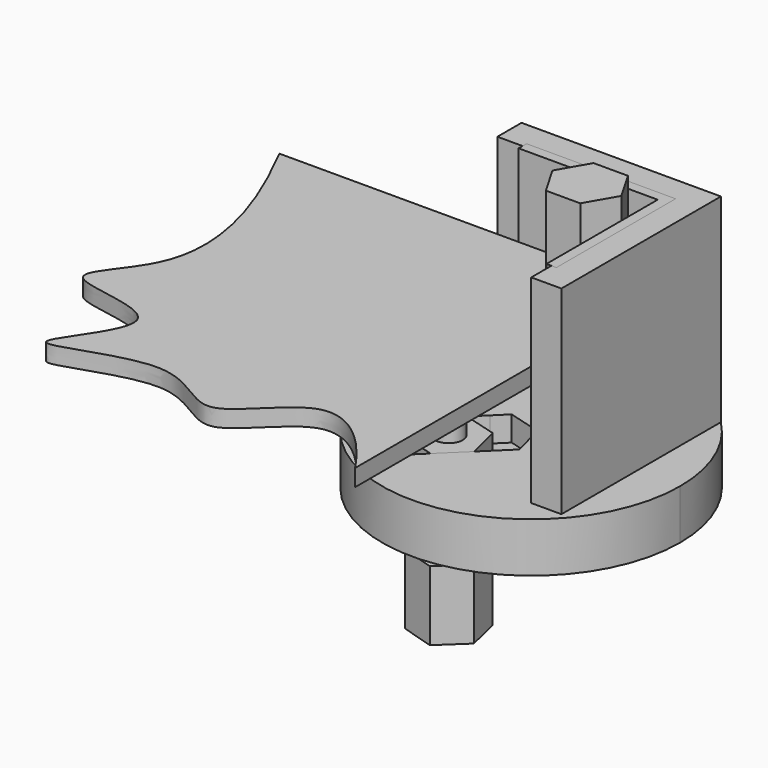
from build123d import *

# Parameters (mm, degrees)
F0_R           = 1.5
F1_DEPTH       = 5
F2_DEPTH       = 20
F3_DEPTH       = 20
F3_DEPTH_BACK  = 2
F4_R           = 1.5
F5_DEPTH       = 2.5
F6_DEPTH       = 2.5
F8_R           = 1.5
F9_DEPTH       = 1.7
F10_R          = 1.4
F11_DEPTH      = 2.5
F12_R          = 1.4
F13_DEPTH      = 10
F13_DEPTH_BACK = 3
F14_R          = 1.4
F15_DEPTH      = 7
F16_DEPTH      = 2.5
F17_R          = 1.5
F18_DEPTH      = 3
F18_DEPTH_BACK = 16.75
F19_R          = 1.5
F20_DEPTH      = 10


with BuildPart() as f1:
    # F0 (on Top) → F1 (new body)
    with BuildSketch(Plane.XY):
        with BuildLine():
            ThreePointArc((10.687071432, 10.524628764), (-13.8805169163, -5.6875808488), (14.9995543431, -0.0004355339))
            ThreePointArc((14.9995543431, -0.0004355339), (13.8796256025, 5.686709781), (10.687071432, 10.524628764))
        make_face()
        Polygon((-0.0255517784, -4.2197033239), (-5.031831142, -9.1122657337), (-6.2705640298, -10.3228609727), (-9.6061093789, -9.387907913), (-10.4641889525, -6.0317643753), (-9.2254560647, -4.8211691363), (-4.2191767011, 0.0713932735), (-2.9804438133, 1.2819885125), (0.3551015358, 0.3470354528), (1.2131811094, -3.0091080849), align=None, mode=Mode.SUBTRACT)
        Polygon((-9.3843074214, 10.524628764), (10.687071432, 10.524628764), (10.687071432, -9.5467500894), (7.6513820053, -9.5467500894), (7.6513820053, -7.0110606627), (7.1513820053, -7.0110606627), (7.1513820053, 6.9889393373), (-6.8486179947, 6.9889393373), (-6.8486179947, 7.4889393373), (-9.3843074214, 7.4889393373), align=None, mode=Mode.SUBTRACT)
        with Locations((3.1513820053, 3.0797987924)):
            Circle(F0_R, mode=Mode.SUBTRACT)
        Polygon((10.687071432, -9.5467500894), (10.687071432, 10.524628764), (-9.3843074214, 10.524628764), (-9.3843074214, 7.4889393373), (-6.8486179947, 7.4889393373), (-6.8486179947, 7.9889393373), (8.1513820053, 7.9889393373), (8.1513820053, -7.0110606627), (7.6513820053, -7.0110606627), (7.6513820053, -9.5467500894), align=None)
        Polygon((-6.2705640298, -10.3228609727), (-5.031831142, -9.1122657337), (-0.0255517784, -4.2197033239), (1.2131811094, -3.0091080849), (0.3551015358, 0.3470354528), (-2.9804438133, 1.2819885125), (-4.2191767011, 0.0713932735), (-9.2254560647, -4.8211691363), (-10.4641889525, -6.0317643753), (-9.6061093789, -9.387907913), align=None)
        with BuildLine():
            Line((-8.177049834, -5.8939432857), (-3.1707704704, -1.0013808758))
            ThreePointArc((-3.1707704704, -1.0013808758), (-1.0495900904, -1.0257487945), (-1.0739580091, -3.1469291745))
            Line((-1.0739580091, -3.1469291745), (-6.0802373727, -8.0394915843))
            ThreePointArc((-6.0802373727, -8.0394915843), (-8.2014177527, -8.0151236657), (-8.177049834, -5.8939432857))
        make_face(mode=Mode.SUBTRACT)
        Polygon((7.1513820053, -7.0110606627), (7.6513820053, -7.0110606627), (8.1513820053, -7.0110606627), (8.1513820053, 7.9889393373), (-6.8486179947, 7.9889393373), (-6.8486179947, 7.4889393373), (-6.8486179947, 6.9889393373), (7.1513820053, 6.9889393373), align=None)
    extrude(amount=-F1_DEPTH)

    # F0 (on Top) → F2 (join)
    with BuildSketch(Plane.XY):
        Polygon((10.687071432, -9.5467500894), (10.687071432, 10.524628764), (-9.3843074214, 10.524628764), (-9.3843074214, 7.4889393373), (-6.8486179947, 7.4889393373), (-6.8486179947, 7.9889393373), (8.1513820053, 7.9889393373), (8.1513820053, -7.0110606627), (7.6513820053, -7.0110606627), (7.6513820053, -9.5467500894), align=None)
    extrude(amount=F2_DEPTH)

    # F4 (on face) → F5 (cut)
    with BuildSketch(Plane(origin=(0, 0, -5), x_dir=(1, 0, 0), z_dir=(0, 0, -1))):
        Polygon((4.0705160108, -6.4197378158), (6.5034210494, -3.9537749058), (5.5842870439, -0.6138358825), (2.2322479998, 0.260140231), (-0.2006570388, -2.2058226789), (0.7184769667, -5.5457617023), align=None)
        with Locations((3.1513820053, -3.0797987924)):
            Circle(F4_R, mode=Mode.SUBTRACT)
    extrude(amount=-F5_DEPTH, mode=Mode.SUBTRACT)

    # F0 (on Top) → F6 (cut)
    with BuildSketch(Plane.XY):
        Polygon((-6.2705640298, -10.3228609727), (-5.031831142, -9.1122657337), (-0.0255517784, -4.2197033239), (1.2131811094, -3.0091080849), (0.3551015358, 0.3470354528), (-2.9804438133, 1.2819885125), (-4.2191767011, 0.0713932735), (-9.2254560647, -4.8211691363), (-10.4641889525, -6.0317643753), (-9.6061093789, -9.387907913), align=None)
        with BuildLine():
            Line((-8.177049834, -5.8939432857), (-3.1707704704, -1.0013808758))
            ThreePointArc((-3.1707704704, -1.0013808758), (-1.0495900904, -1.0257487945), (-1.0739580091, -3.1469291745))
            Line((-1.0739580091, -3.1469291745), (-6.0802373727, -8.0394915843))
            ThreePointArc((-6.0802373727, -8.0394915843), (-8.2014177527, -8.0151236657), (-8.177049834, -5.8939432857))
        make_face(mode=Mode.SUBTRACT)
    extrude(amount=-F6_DEPTH, mode=Mode.SUBTRACT)


with BuildPart() as f3:
    # F0 (on Top) → F3 (new body, two sides)
    with BuildSketch(Plane.XY) as f3_sk:
        Polygon((7.1513820053, -7.0110606627), (7.6513820053, -7.0110606627), (8.1513820053, -7.0110606627), (8.1513820053, 7.9889393373), (-6.8486179947, 7.9889393373), (-6.8486179947, 7.4889393373), (-6.8486179947, 6.9889393373), (7.1513820053, 6.9889393373), align=None)
    extrude(amount=F3_DEPTH)
    extrude(f3_sk.sketch, amount=-F3_DEPTH_BACK)


with BuildPart() as f9:
    # F8 (on offset) → F9 (new body)
    with BuildSketch(Plane.XY.offset(10)):
        with BuildLine():
            Line((7.1513820053, -31.09319371), (7.1513820053, 6.9889393373))
            Line((7.1513820053, 6.9889393373), (-30.9342486239, 6.9889393373))
            add(Edge.make_bspline(
                [(-30.9342486239, 6.9889393373), (-27.2519677157, -0.1294210952), (-22.7293333964, -12.1300855711), (-34.0610705435, -20.5501134131), (-16.9446822387, -19.7516150943), (-30.1997724877, -33.3386646834), (-14.1696809036, -24.3767968124), (-8.1671886312, -33.3553621754), (-1.2568024422, -21.3864704219), (4.7130379425, -27.413404081), (7.1513820053, -31.09319371)],
                knots=[0, 0, 0, 0, 0.1804825249, 0.2871406378, 0.402609914, 0.5159111982, 0.6429904922, 0.7542061529, 0.8712630993, 1, 1, 1, 1], degree=3))
        make_face()
        with Locations((3.1513820053, 3.0797987924)):
            Circle(F8_R, mode=Mode.SUBTRACT)
    extrude(amount=F9_DEPTH)


with BuildPart() as f11:
    # F10 (on face) → F11 (new body, through all)
    with BuildSketch(Plane.XY):
        Polygon((-3.7930982542, -7.9016704947), (-1.3156324786, -5.4804800167), (-2.1737120521, -2.124336479), (-5.5092574013, -1.1893834193), (-7.9867231769, -3.6105738973), (-7.1286436033, -6.966717435), align=None)
        with Locations((-4.6511778277, -4.545526957)):
            Circle(F10_R, mode=Mode.SUBTRACT)
    extrude(amount=-F11_DEPTH)


with BuildPart() as f13:
    # F12 (on face) → F13 (new body, two sides)
    with BuildSketch(Plane.XY) as f13_sk:
        with Locations((-4.6511778277, -4.545526957)):
            Circle(F12_R)
    extrude(amount=-F13_DEPTH)
    extrude(f13_sk.sketch, amount=F13_DEPTH_BACK)


with BuildPart() as f15:
    # F14 (on face) → F15 (new body)
    with BuildSketch(Plane(origin=(0, 0, -10), x_dir=(1, 0, 0), z_dir=(0, 0, -1))):
        Polygon((-1.3332408629, 5.5411645906), (-3.854456829, 7.9167634735), (-7.1723937938, 6.9211258399), (-7.9691147926, 3.5498893234), (-5.4478988265, 1.1742904405), (-2.1299618617, 2.1699280741), align=None)
        with Locations((-4.6511778277, 4.545526957)):
            Circle(F14_R, mode=Mode.SUBTRACT)
    extrude(amount=F15_DEPTH)


with BuildPart() as f16:
    # F16 (new, through all): a face of the model
    f16_faces = [f1.part.faces().sort_by_distance(p)[0] for p in [
        (2.4183734556, 5.8911722846, -2.5),
    ]]
    extrude(f16_faces, amount=F16_DEPTH)


with BuildPart() as f18:
    # F17 (on face) → F18 (new body, two sides)
    with BuildSketch(Plane(origin=(0, 0, -5), x_dir=(1, 0, 0), z_dir=(0, 0, -1))) as f18_sk:
        with Locations((3.1513820053, -3.0797987924)):
            Circle(F17_R)
    extrude(amount=F18_DEPTH)
    extrude(f18_sk.sketch, amount=-F18_DEPTH_BACK)

    # F19 (on face) → F20 (join)
    with BuildSketch(Plane.XY.offset(11.75)):
        Polygon((1.4193311978, 0.0797987924), (4.8834328129, 0.0797987924), (6.6154836205, 3.0797987924), (4.8834328129, 6.0797987924), (1.4193311978, 6.0797987924), (-0.3127196098, 3.0797987924), align=None)
        with Locations((3.1513820053, 3.0797987924)):
            Circle(F19_R, mode=Mode.SUBTRACT)
        with Locations((3.1513820053, 3.0797987924)):
            Circle(F19_R)
    extrude(amount=F20_DEPTH)


with BuildPart() as f1_1:
    add(f1.part)

    # F21: cut F3
    add(f3.part, mode=Mode.SUBTRACT)


solid = Compound([f3.part, f9.part, f11.part, f13.part, f15.part, f16.part, f18.part, f1_1.part])
